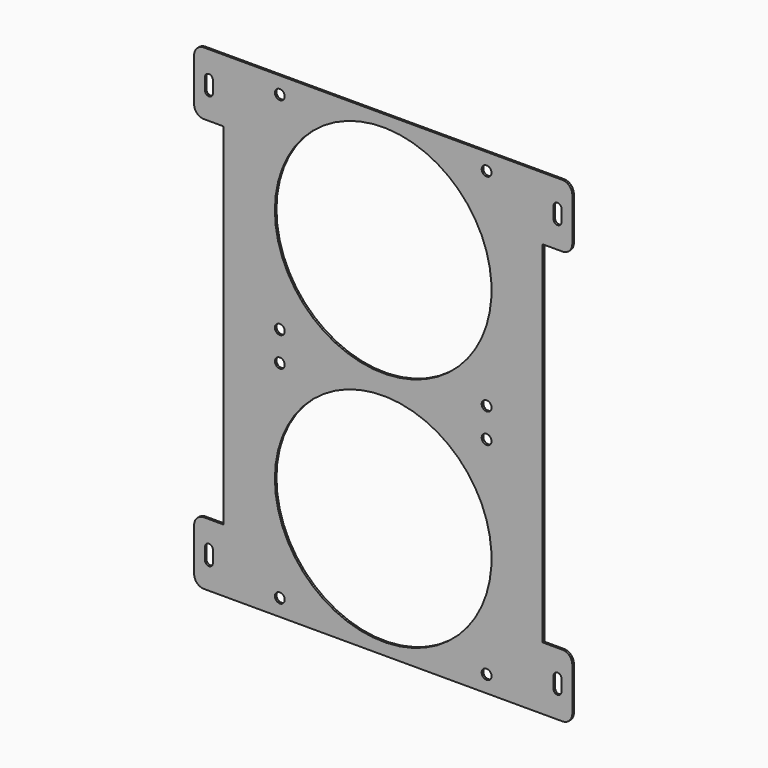
from build123d import *

# Parameters (mm, degrees)
F0_W      = 192
F0_H      = 242
F1_DEPTH  = 1
F3_D      = 110
F5_D      = 5
F6_W      = 15
F6_H      = 178
F7_DEPTH  = 1
F8_R      = 5
F9_W      = 4
F9_H      = 10
F10_DEPTH = 1
F11_R     = 1.99999


# Not quite as in the source:
# - a fillet or chamfer is up to 0.001 mm smaller than in the source, because OpenCascade refuses the exact size


with BuildPart() as f1:
    # F0 (on Front) → F1 (new body)
    with BuildSketch(Plane.XZ):
        with Locations((96, 121)):
            Rectangle(F0_W, F0_H)
    extrude(amount=F1_DEPTH)

    # F3 (through all)
    with Locations(Plane.XZ.offset(1)):
        with Locations((96, 181), (96, 61)):
            Hole(F3_D / 2)

    # F5 (through all)
    with Locations(Plane.XZ.offset(1)):
        with Locations((43.5, 233.5), (148.5, 233.5), (43.5, 128.5), (148.5, 128.5), (43.5, 113.5), (148.5, 113.5), (43.5, 8.5), (148.5, 8.5)):
            Hole(F5_D / 2)

    # F6 (on face) → F7 (cut)
    with BuildSketch(Plane.XZ.offset(1)):
        with Locations((7.5, 121)):
            Rectangle(F6_W, F6_H)
        with Locations((184.5, 121)):
            Rectangle(F6_W, F6_H)
    extrude(amount=-F7_DEPTH, mode=Mode.SUBTRACT)

    # F8
    f8_edges = [f1.edges().sort_by_distance(p)[0] for p in [
        (0, -0.5, 210),
        (0, -0.5, 242),
        (0, -0.5, 32),
        (0, -0.5, 0),
        (192, -0.5, 32),
        (192, -0.5, 0),
        (192, -0.5, 242),
        (192, -0.5, 210),
    ]]
    fillet(f8_edges, radius=F8_R)

    # F9 (on face) → F10 (cut)
    with BuildSketch(Plane.XZ.offset(1)):
        with Locations((7.5, 226)):
            Rectangle(F9_W, F9_H)
        with Locations((184.5, 226)):
            Rectangle(F9_W, F9_H)
        with Locations((7.5, 16)):
            Rectangle(F9_W, F9_H)
        with Locations((184.5, 16)):
            Rectangle(F9_W, F9_H)
    extrude(amount=-F10_DEPTH, mode=Mode.SUBTRACT)

    # F11 (radius 2 in the source; OpenCascade refuses exactly that, so slightly less here)
    f11_edges = [f1.edges().sort_by_distance(p)[0] for p in [
        (9.5, -0.5, 231),
        (5.5, -0.5, 231),
        (5.5, -0.5, 221),
        (9.5, -0.5, 221),
        (182.5, -0.5, 231),
        (186.5, -0.5, 231),
        (182.5, -0.5, 221),
        (186.5, -0.5, 221),
        (182.5, -0.5, 21),
        (186.5, -0.5, 21),
        (186.5, -0.5, 11),
        (182.5, -0.5, 11),
        (5.5, -0.5, 21),
        (9.5, -0.5, 21),
        (9.5, -0.5, 11),
        (5.5, -0.5, 11),
    ]]
    fillet(f11_edges, radius=F11_R)


solid = f1.part
